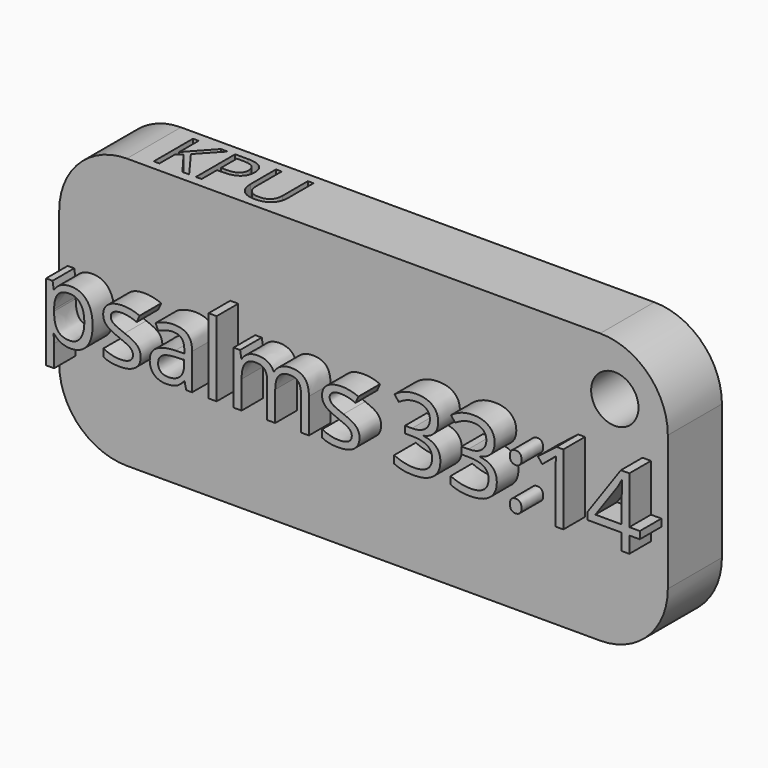
from build123d import *

# Parameters (mm, degrees)
F0_W         = 45
F0_H         = 20
F1_DEPTH     = 5
F2_TEXT_SIZE = 7.3007503549
F3_DEPTH     = 2
F4_R         = 5
F5_TEXT_SIZE = 5.0815392266
F6_DEPTH     = 2
F7_R         = 1.75
F8_DEPTH     = 5


# Not quite as in the source:
# - Text() gives the source's letters only with a copy of the font that has no kerning and outlines rounded to 1/6400 em; it was checked with that copy


with BuildPart() as f1:
    # F0 (on Front) → F1 (new body)
    with BuildSketch(Plane.XZ):
        with Locations((22.5, 10)):
            Rectangle(F0_W, F0_H)
    extrude(amount=F1_DEPTH)

    # F2 (on face) → F3 (join)
    with BuildSketch(Plane.XZ.offset(5)):
        with Locations((2.3865e-06, 7.6854927465)):
            Text('psalms 33:14', F2_TEXT_SIZE, font='Open Sans', text_align=(TextAlign.LEFT, TextAlign.BOTTOM))
    extrude(amount=F3_DEPTH)

    # F4
    f4_edges = [f1.edges().sort_by_distance(p)[0] for p in [
        (0, -2.5, 20),
        (45, -2.5, 20),
        (45, -2.5, 0),
        (0, -2.5, 0),
    ]]
    fillet(f4_edges, radius=F4_R)

    # F5 (on face) → F6 (cut)
    with BuildSketch(Plane.XY.offset(20)):
        with Locations((5.9306225739, -4.3047419749)):
            Text('KPU', F5_TEXT_SIZE, font='Open Sans', text_align=(TextAlign.LEFT, TextAlign.BOTTOM))
    extrude(amount=-F6_DEPTH, mode=Mode.SUBTRACT)

    # F7 (on face) → F8 (cut)
    with BuildSketch(Plane.XZ.offset(5)):
        with Locations((41.0805240744, 16.0843612615)):
            Circle(F7_R)
    extrude(amount=-F8_DEPTH, mode=Mode.SUBTRACT)


solid = f1.part
